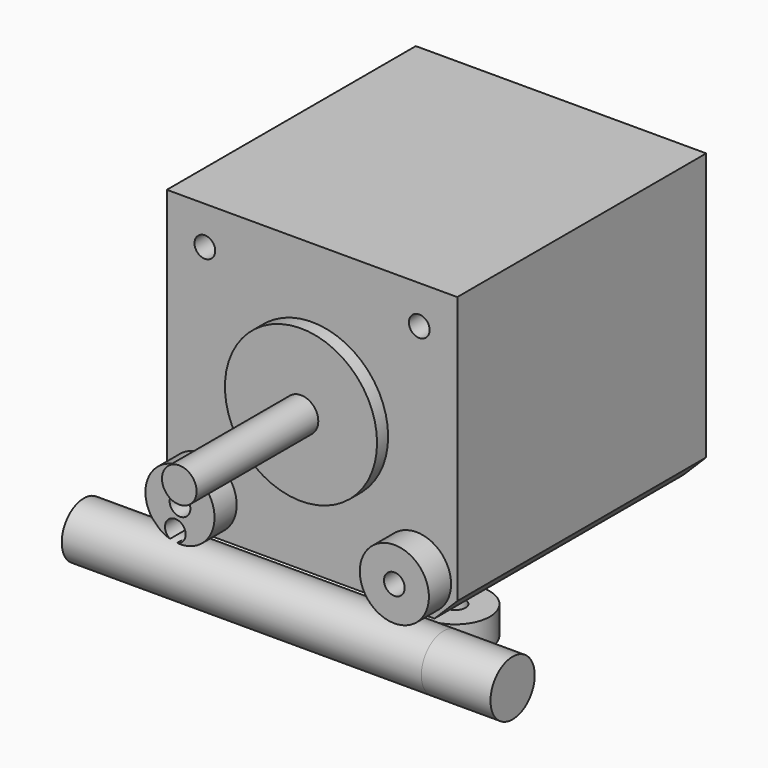
from build123d import *

# Parameters (mm, degrees)
F0_R          = 5
F0_R_2        = 1.5
F0_R_3        = 11
F0_R_4        = 2.5
F1_DEPTH      = 45
F2_DEPTH      = 2
F3_DEPTH      = 24
F4_START      = 0.5
F4_DEPTH      = 4
F5_R          = 4
F6_DEPTH      = 52
F6_DEPTH_BACK = 10
F7_ANGLE      = -90
F8_SIZE       = 3.3


# Not quite as in the source:
# - a feature names something its author has since deleted; it is built from what else it names


with BuildPart() as f1:
    # F0 (on Front) → F1 (new body)
    with BuildSketch(Plane.XZ):
        with BuildLine():
            Line((21, 21), (-21, 21))
            Line((-21, 21), (-21, -17))
            Line((-21, -17), (-19.5, -18.5))
            ThreePointArc((-19.5, -18.5), (-17.0811388301, -10.7565835097), (-10.5, -15.5))
            ThreePointArc((-10.5, -15.5), (-12.1214833592, -19.1858683248), (-15.9342501231, -20.4811069885))
            ThreePointArc((-15.9342501231, -20.4811069885), (-16.454233474, -20.4731269415), (-16.9402414775, -20.2880794152))
            ThreePointArc((-16.9402414775, -20.2880794152), (-17.7548178165, -19.9627118005), (-18.5, -19.5))
            Line((-18.5, -19.5), (-17, -21))
            Line((-17, -21), (21, -21))
            Line((21, -21), (21, 21))
        make_face()
        with Locations((15.5, -15.5)):
            Circle(F0_R, mode=Mode.SUBTRACT)
        with Locations((-15.5, 15.5)):
            Circle(F0_R_2, mode=Mode.SUBTRACT)
        Circle(F0_R_3, mode=Mode.SUBTRACT)
        with Locations((15.5, 15.5)):
            Circle(F0_R_2, mode=Mode.SUBTRACT)
        Circle(F0_R_3)
        Circle(F0_R_4, mode=Mode.SUBTRACT)
        with Locations((15.5, -15.5)):
            Circle(F0_R)
        with Locations((15.5, -15.5)):
            Circle(F0_R_2, mode=Mode.SUBTRACT)
        with BuildLine():
            ThreePointArc((-10.5, -15.5), (-17.0811388301, -10.7565835097), (-19.5, -18.5))
            Line((-19.5, -18.5), (-18.5, -19.5))
            ThreePointArc((-18.5, -19.5), (-17.7548178165, -19.9627118005), (-16.9402414775, -20.2880794152))
            ThreePointArc((-16.9402414775, -20.2880794152), (-16.9121797536, -17.6955838656), (-14.6715728753, -19))
            ThreePointArc((-14.6715728753, -19), (-15.0300860973, -19.9731433275), (-15.9342501231, -20.4811069885))
            ThreePointArc((-15.9342501231, -20.4811069885), (-12.1214833592, -19.1858683248), (-10.5, -15.5))
        make_face()
        with Locations((-15.5, -15.5)):
            Circle(F0_R_2, mode=Mode.SUBTRACT)
        Circle(F0_R_4)
        with BuildLine():
            Line((-19.5, -18.5), (-21, -17))
            Line((-21, -17), (-21, -21))
            Line((-21, -21), (-17, -21))
            Line((-17, -21), (-18.5, -19.5))
            ThreePointArc((-18.5, -19.5), (-19.0355339059, -19.0355339059), (-19.5, -18.5))
        make_face()
    extrude(amount=-F1_DEPTH)

    # F0 (on Front) → F2 (join)
    with BuildSketch(Plane.XZ):
        Circle(F0_R_3)
        Circle(F0_R_4, mode=Mode.SUBTRACT)
    extrude(amount=F2_DEPTH)

    # F0 (on Front) → F3 (join)
    with BuildSketch(Plane.XZ):
        Circle(F0_R_4)
    extrude(amount=F3_DEPTH)

    # F8
    f8_edges = [f1.edges().sort_by_distance(p)[0] for p in [
        (21, 22.5, -21),
    ]]
    chamfer(f8_edges, length=F8_SIZE)


with BuildPart() as f4:
    # F0 (on Front) → F4 (new body)
    with BuildSketch(Plane.XZ.offset(F4_START)):
        with BuildLine():
            ThreePointArc((-10.5, -15.5), (-17.0811388301, -10.7565835097), (-19.5, -18.5))
            Line((-19.5, -18.5), (-18.5, -19.5))
            ThreePointArc((-18.5, -19.5), (-17.7548178165, -19.9627118005), (-16.9402414775, -20.2880794152))
            ThreePointArc((-16.9402414775, -20.2880794152), (-16.9121797536, -17.6955838656), (-14.6715728753, -19))
            ThreePointArc((-14.6715728753, -19), (-15.0300860973, -19.9731433275), (-15.9342501231, -20.4811069885))
            ThreePointArc((-15.9342501231, -20.4811069885), (-12.1214833592, -19.1858683248), (-10.5, -15.5))
        make_face()
        with Locations((-15.5, -15.5)):
            Circle(F0_R_2, mode=Mode.SUBTRACT)
    extrude(amount=F4_DEPTH)


with BuildPart() as f4b:
    # F0 (on Front) → F4, piece 2 (new body)
    with BuildSketch(Plane.XZ.offset(F4_START)):
        with Locations((15.5, -15.5)):
            Circle(F0_R)
        with Locations((15.5, -15.5)):
            Circle(F0_R_2, mode=Mode.SUBTRACT)
    extrude(amount=F4_DEPTH)


with BuildPart() as f6:
    # F5 (on face) → F6 (new body, two sides)
    with BuildSketch(Plane.YZ.offset(21)) as f6_sk:
        with Locations((-2.5, -24.5)):
            Circle(F5_R)
    extrude(amount=-F6_DEPTH)
    extrude(f6_sk.sketch, amount=F6_DEPTH_BACK)


with BuildPart() as f7_1:
    # F7: copy of F4b
    add(f4b.part.rotate(Axis((21, -2.5, -24.5), (1, 0, 0)), F7_ANGLE))


solid = Compound([f1.part, f4.part, f4b.part, f6.part, f7_1.part])
